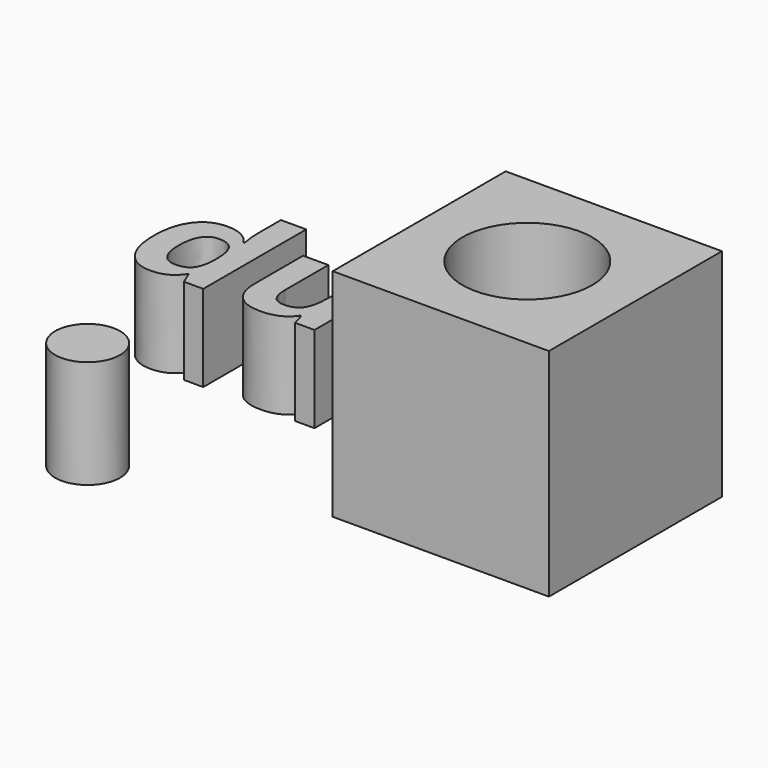
from build123d import *

# Parameters (mm, degrees)
F0_W         = 50
F0_H         = 50
F0_R         = 15
F1_DEPTH     = 50
F2_TEXT_SIZE = 39.1789893102
F3_DEPTH     = 20
F4_R         = 7.5
F5_DEPTH     = 25
F6_R         = 6.5
F7_DEPTH     = 23


# Not quite as in the source:
# - Text() gives the source's letters only with a copy of the font that has no kerning and outlines rounded to 1/6400 em; it was checked with that copy


with BuildPart() as f1:
    # F0 (on Top) → F1 (new body)
    with BuildSketch(Plane.XY):
        Rectangle(F0_W, F0_H)
        Circle(F0_R, mode=Mode.SUBTRACT)
    extrude(amount=F1_DEPTH)


with BuildPart() as f3:
    # F2 (on Top) → F3 (new body)
    with BuildSketch(Plane.XY):
        with Locations((-96.6850593686, 0)):
            Text('du', F2_TEXT_SIZE, font='Open Sans', font_style=FontStyle.BOLD, text_align=(TextAlign.LEFT, TextAlign.BOTTOM))
    extrude(amount=F3_DEPTH)


with BuildPart() as f5:
    # F4 (on Top) → F5 (new body)
    with BuildSketch(Plane.XY):
        with Locations((-71.994587779, -37.0922721922)):
            Circle(F4_R)
    extrude(amount=F5_DEPTH)

    # F6 (on Top) → F7 (cut)
    with BuildSketch(Plane.XY):
        with Locations((-72.0235258341, -36.9147434831)):
            Circle(F6_R)
    extrude(amount=F7_DEPTH, mode=Mode.SUBTRACT)


solid = Compound([f1.part, f3.part, f5.part])
